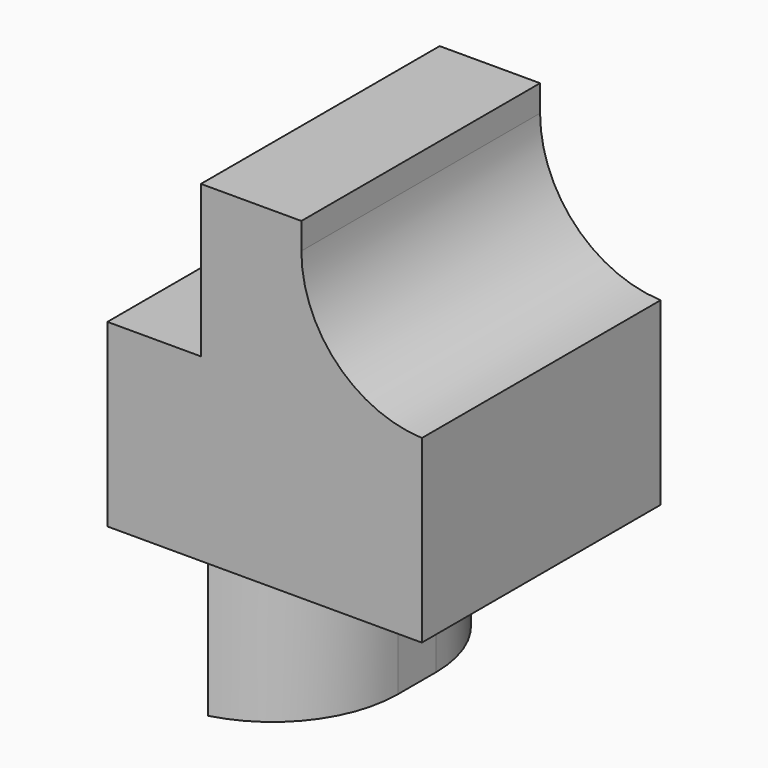
from build123d import *

# Parameters (mm, degrees)
F0_W        = 31.884431839
F0_H        = 48.2252053916
F0_W_2      = 29.4931009412
F0_H_2      = 43.4425398707
F1_DEPTH    = 94.742
F2_R        = 5.08
F3_T1_DEPTH = 94.742
F3_T3_DEPTH = 143.0892046577


# Not quite as in the source:
# - a fillet or chamfer that OpenCascade refuses, or shapes differently, is made with other operations: its cross-section is extruded or revolved along the edge and cut away or added


with BuildPart() as f1:
    # F0 (on Front) → F1 (new body)
    with BuildSketch(Plane.XZ):
        Polygon((-15.9422159195, 31.5855164081), (-45.6345975399, 31.5855164081), (-45.6345975399, -25.6071873009), (-14.7465504706, -25.6071873009), (14.7465504706, -25.6071873009), (54.2035363615, -25.6071873009), (54.2035363615, 31.5855164081), (15.9422159195, 31.5855164081), align=None)
        with Locations((0, 55.6981191039)):
            Rectangle(F0_W, F0_H)
        with Locations((0, -47.3284572363)):
            Rectangle(F0_W_2, F0_H_2)
    extrude(amount=F1_DEPTH)

    # F2
    f2_edges = [f1.edges().sort_by_distance(p)[0] for p in [
        (-30.788407, 0, 31.585516),
    ]]
    fillet(f2_edges, radius=F2_R)

    # F3: fillet of radius 39.8586659148 on 3 edges, made by hand

    # F3_s2 → F3_t1 (join)
    with BuildSketch(Plane.XZ):
        with BuildLine():
            ThreePointArc((54.2035363615, 31.5855164081), (27.0573494482, 43.798350801), (15.9422159195, 71.4121624625))
            Line((15.9422159195, 71.4121624625), (15.9422159195, 31.5855164081))
            Line((15.9422159195, 31.5855164081), (54.2035363615, 31.5855164081))
        make_face()
    extrude(amount=F3_T1_DEPTH)

    # F3_s4 → F3_t3 (cut)
    with BuildSketch(Plane.XY.offset(-168.6963919586)):
        with BuildLine():
            ThreePointArc((14.7465504706, -39.8586659148), (3.0722175132, -11.6743329574), (-25.1121154442, 0))
            Line((-25.1121154442, 0), (14.7465504706, 0))
            Line((14.7465504706, 0), (14.7465504706, -39.8586659148))
        make_face()
        with BuildLine():
            ThreePointArc((14.7465504706, -54.8833340852), (3.0722175132, -83.0676670426), (-25.1121154442, -94.742))
            Line((-25.1121154442, -94.742), (14.7465504706, -94.742))
            Line((14.7465504706, -94.742), (14.7465504706, -54.8833340852))
        make_face()
    extrude(amount=F3_T3_DEPTH, mode=Mode.SUBTRACT)


solid = f1.part
